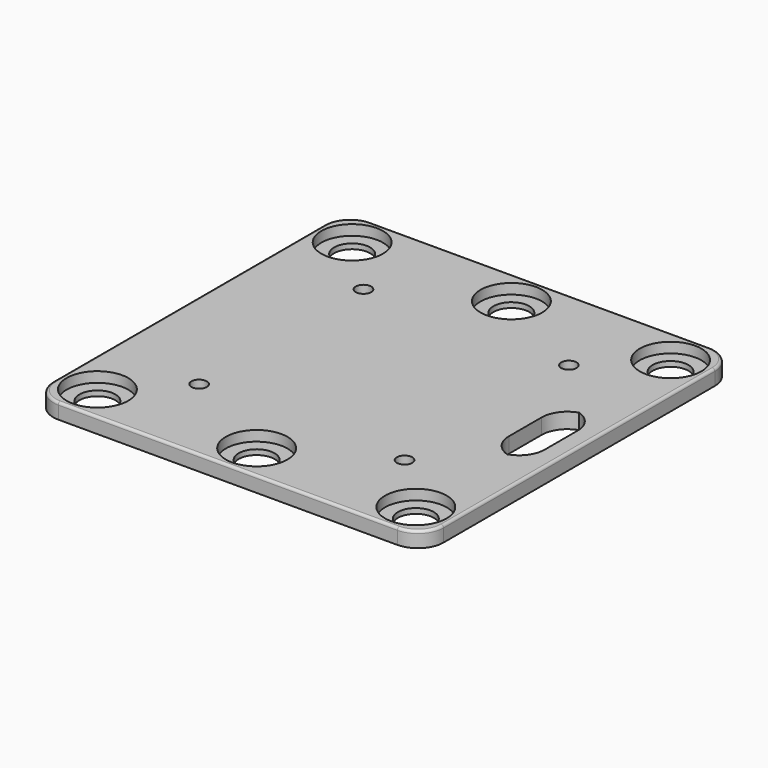
from build123d import *

# Parameters (mm, degrees)
F0_W        = 76
F0_H        = 76
F0_R        = 6
F0_R_2      = 1.5
F0_W_2      = 7
F0_H_2      = 18
F1_DEPTH    = 3
F0_R_3      = 3.5
F2_DEPTH    = 1
F3_T1_DEPTH = 3
F3_T3_DEPTH = 28
F4_R        = 0.5


# Not quite as in the source:
# - a fillet or chamfer that OpenCascade refuses, or shapes differently, is made with other operations: its cross-section is extruded or revolved along the edge and cut away or added
# - a feature names something its author has since deleted; it is built from what else it names


with BuildPart() as f1:
    # F0 (on Top) → F1 (new body)
    with BuildSketch(Plane.XY):
        Rectangle(F0_W, F0_H)
        with Locations((-31, -31)):
            Circle(F0_R, mode=Mode.SUBTRACT)
        with Locations((-20, -20)):
            Circle(F0_R_2, mode=Mode.SUBTRACT)
        with Locations((0, -31)):
            Circle(F0_R, mode=Mode.SUBTRACT)
        with Locations((31, -31)):
            Circle(F0_R, mode=Mode.SUBTRACT)
        with Locations((20, -20)):
            Circle(F0_R_2, mode=Mode.SUBTRACT)
        with Locations((-20, 20)):
            Circle(F0_R_2, mode=Mode.SUBTRACT)
        with Locations((-31, 31)):
            Circle(F0_R, mode=Mode.SUBTRACT)
        with Locations((31, 0)):
            Rectangle(F0_W_2, F0_H_2, mode=Mode.SUBTRACT)
        with Locations((0, 31)):
            Circle(F0_R, mode=Mode.SUBTRACT)
        with Locations((20, 20)):
            Circle(F0_R_2, mode=Mode.SUBTRACT)
        with Locations((31, 31)):
            Circle(F0_R, mode=Mode.SUBTRACT)
    extrude(amount=F1_DEPTH)

    # F0 (on Top) → F2 (join)
    with BuildSketch(Plane.XY):
        with Locations((-31, 31)):
            Circle(F0_R)
        with Locations((-31, 31)):
            Circle(F0_R_3, mode=Mode.SUBTRACT)
        with Locations((31, 31)):
            Circle(F0_R)
        with Locations((31, 31)):
            Circle(F0_R_3, mode=Mode.SUBTRACT)
        with Locations((31, -31)):
            Circle(F0_R)
        with Locations((31, -31)):
            Circle(F0_R_3, mode=Mode.SUBTRACT)
        with Locations((-31, -31)):
            Circle(F0_R)
        with Locations((-31, -31)):
            Circle(F0_R_3, mode=Mode.SUBTRACT)
        with Locations((0, 31)):
            Circle(F0_R)
        with Locations((0, 31)):
            Circle(F0_R_3, mode=Mode.SUBTRACT)
        with Locations((0, -31)):
            Circle(F0_R)
        with Locations((0, -31)):
            Circle(F0_R_3, mode=Mode.SUBTRACT)
    extrude(amount=F2_DEPTH)

    # F3: fillet of radius 5 on 8 edges, made by hand

    # F3_s2 → F3_t1 (join)
    with BuildSketch(Plane.XY):
        with BuildLine():
            ThreePointArc((29.5, 9), (33.0355339059, 7.5355339059), (34.5, 4))
            Line((34.5, 4), (34.5, 9))
            Line((34.5, 9), (29.5, 9))
        make_face()
        with BuildLine():
            ThreePointArc((29.5, -9), (33.0355339059, -7.5355339059), (34.5, -4))
            Line((34.5, -4), (34.5, -9))
            Line((34.5, -9), (29.5, -9))
        make_face()
        with BuildLine():
            ThreePointArc((32.5, -9), (28.9644660941, -7.5355339059), (27.5, -4))
            Line((27.5, -4), (27.5, -9))
            Line((27.5, -9), (32.5, -9))
        make_face()
        with BuildLine():
            ThreePointArc((27.5, 4), (28.9644660941, 7.5355339059), (32.5, 9))
            Line((32.5, 9), (27.5, 9))
            Line((27.5, 9), (27.5, 4))
        make_face()
    extrude(amount=F3_T1_DEPTH)

    # F3_s4 → F3_t3 (cut)
    with BuildSketch(Plane.XY.offset(-12.5)):
        with BuildLine():
            ThreePointArc((-33, -38), (-36.5355339059, -36.5355339059), (-38, -33))
            Line((-38, -33), (-38, -38))
            Line((-38, -38), (-33, -38))
        make_face()
        with BuildLine():
            ThreePointArc((33, -38), (36.5355339059, -36.5355339059), (38, -33))
            Line((38, -33), (38, -38))
            Line((38, -38), (33, -38))
        make_face()
        with BuildLine():
            ThreePointArc((38, 33), (36.5355339059, 36.5355339059), (33, 38))
            Line((33, 38), (38, 38))
            Line((38, 38), (38, 33))
        make_face()
        with BuildLine():
            ThreePointArc((-38, 33), (-36.5355339059, 36.5355339059), (-33, 38))
            Line((-33, 38), (-38, 38))
            Line((-38, 38), (-38, 33))
        make_face()
    extrude(amount=F3_T3_DEPTH, mode=Mode.SUBTRACT)

    # F4
    f4_edges = [f1.edges().sort_by_distance(p)[0] for p in [
        (0, -38, 3),
    ]]
    fillet(f4_edges, radius=F4_R)


solid = f1.part
